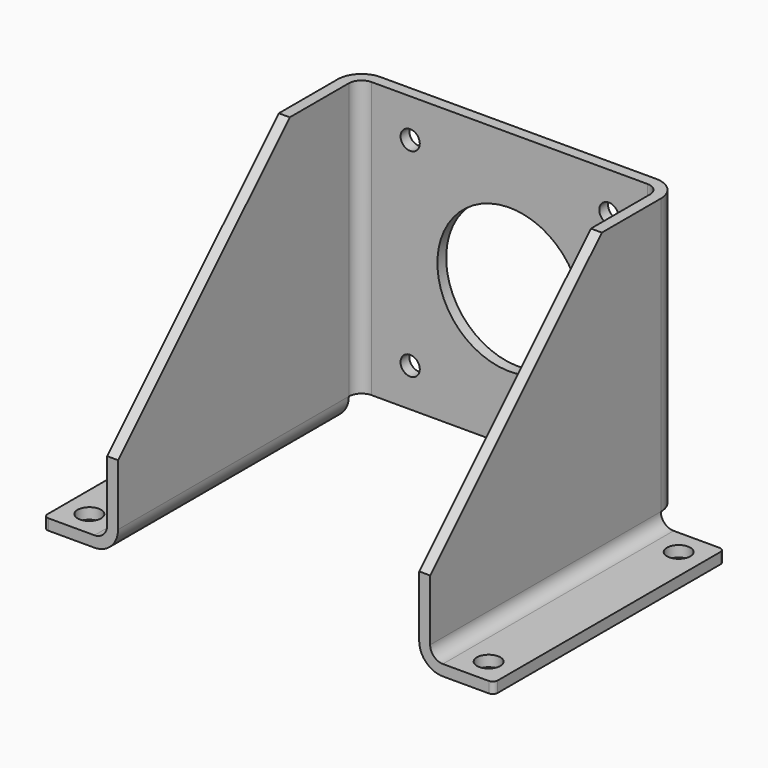
from build123d import *

# Parameters (mm, degrees)
F1_DEPTH  = 43.0059846
F4_DEPTH  = 44.9897246
F5_R      = 1.98374
F6_R      = 3.69316
F7_SIZE   = 33.4809846
F8_R      = 11.2530001
F8_R_2    = 1.5
F9_DEPTH  = 1.70942
F10_R     = 1.8288
F11_DEPTH = 1.70942
F12_R     = 0.762


with BuildPart() as f1:
    # F0 (on Top) → F1 (new body)
    with BuildSketch(Plane.XY):
        Polygon((-1.70942, 0), (0, 0), (0, 46.9734646), (46.9734646, 46.9734646), (46.9734646, 0), (48.6828846, 0), (48.6828846, 48.6828846), (-1.70942, 48.6828846), align=None)
    extrude(amount=F1_DEPTH)

    # F3 (on face) → F4 (join, through all)
    with BuildSketch(Plane.XZ):
        Polygon((48.6828846, 0), (46.9734646, 0), (46.9734646, -3.69316), (58.6041246, -3.69316), (58.6041246, -1.98374), (48.6828846, -1.98374), align=None)
        Polygon((0, 0), (-1.70942, 0), (-1.70942, -1.98374), (-11.63066, -1.98374), (-11.63066, -3.69316), (0, -3.69316), align=None)
    extrude(amount=-F4_DEPTH)

    # F5
    f5_edges = [f1.edges().sort_by_distance(p)[0] for p in [
        (0, 46.973465, 21.502992),
        (46.973465, 46.973465, 21.502992),
        (-1.70942, 22.494862, -1.98374),
        (48.682885, 22.494862, -1.98374),
    ]]
    fillet(f5_edges, radius=F5_R)

    # F6
    f6_edges = [f1.edges().sort_by_distance(p)[0] for p in [
        (48.682885, 48.682885, 21.502992),
        (-1.70942, 48.682885, 21.502992),
        (0, 22.494862, -3.69316),
        (46.973465, 22.494862, -3.69316),
    ]]
    fillet(f6_edges, radius=F6_R)

    # F7
    f7_edges = [f1.edges().sort_by_distance(p)[0] for p in [
        (-0.85471, 0, 43.005985),
        (47.828175, 0, 43.005985),
    ]]
    chamfer(f7_edges, length=F7_SIZE)

    # F8 (on face) → F9 (cut, through all)
    with BuildSketch(Plane.XZ.offset(-46.9734646)):
        with Locations((23.4867323, 21.5029923)):
            Circle(F8_R)
        with Locations((38.9867267, 37.0029867)):
            Circle(F8_R_2)
        with Locations((38.9867267, 6.0029979)):
            Circle(F8_R_2)
        with Locations((7.9867379, 6.0029979)):
            Circle(F8_R_2)
        with Locations((7.9867379, 37.0029867)):
            Circle(F8_R_2)
    extrude(amount=-F9_DEPTH, mode=Mode.SUBTRACT)

    # F10 (on face) → F11 (cut, through all)
    with BuildSketch(Plane(origin=(0, 0, -3.69316), x_dir=(1, 0, 0), z_dir=(0, 0, -1))):
        with Locations((54.6353746, -41.0209746001)):
            Circle(F10_R)
        with Locations((-7.66191, -41.0209746001)):
            Circle(F10_R)
        with Locations((-7.66191, -3.9687499999)):
            Circle(F10_R)
        with Locations((54.6353746, -3.9687499999)):
            Circle(F10_R)
    extrude(amount=-F11_DEPTH, mode=Mode.SUBTRACT)

    # F12
    f12_edges = [f1.edges().sort_by_distance(p)[0] for p in [
        (58.604125, 0, -2.83845),
        (-11.63066, 0, -2.83845),
        (-11.63066, 44.989725, -2.83845),
        (58.604125, 44.989725, -2.83845),
    ]]
    fillet(f12_edges, radius=F12_R)


solid = f1.part
